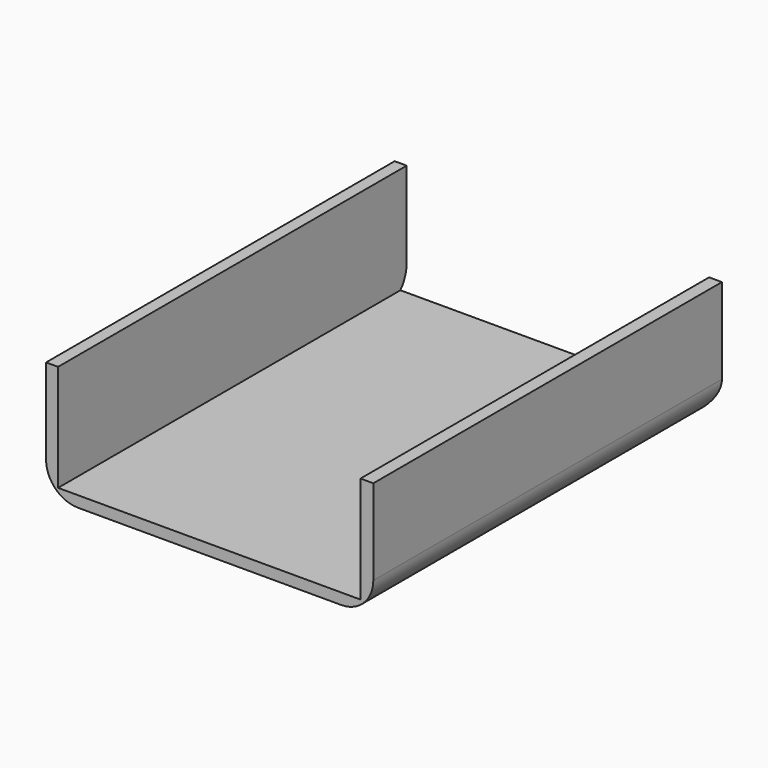
from build123d import *

# Parameters (mm, degrees)
F1_DEPTH    = 34.52499953
F2_T1_DEPTH = 94.44999906
F2_T3_DEPTH = 77.25000044


# Not quite as in the source:
# - a fillet or chamfer that OpenCascade refuses, or shapes differently, is made with other operations: its cross-section is extruded or revolved along the edge and cut away or added


with BuildPart() as f1:
    # F0 (on Front) → F1 (new body, symmetric)
    with BuildSketch(Plane.XZ):
        Polygon((-24.9640439777, 0), (-24.9640439777, -18.630000078), (26.8859564623, -18.630000078), (26.8859564623, 0), (24.8539564623, 0), (24.8539564623, -16.881729), (-23.0624323377, -16.881729), (-23.0624323377, 0), align=None)
    extrude(amount=F1_DEPTH, both=True)

    # F2: fillet of radius 5.08 on 3 edges, made by hand

    # F2_s2 → F2_t1 (cut)
    with BuildSketch(Plane.XZ.offset(-47.22499953)):
        with BuildLine():
            ThreePointArc((26.8859564623, -13.550000078), (25.3980589107, -17.1421025264), (21.8059564623, -18.630000078))
            Line((21.8059564623, -18.630000078), (26.8859564623, -18.630000078))
            Line((26.8859564623, -18.630000078), (26.8859564623, -13.550000078))
        make_face()
        with BuildLine():
            ThreePointArc((-24.9640439777, -13.550000078), (-23.4761464261, -17.1421025264), (-19.8840439777, -18.630000078))
            Line((-19.8840439777, -18.630000078), (-24.9640439777, -18.630000078))
            Line((-24.9640439777, -18.630000078), (-24.9640439777, -13.550000078))
        make_face()
    extrude(amount=F2_T1_DEPTH, mode=Mode.SUBTRACT)

    # F2_s4 → F2_t3 (cut)
    with BuildSketch(Plane.YZ.offset(-37.6640439777)):
        with BuildLine():
            ThreePointArc((29.44499953, -18.630000078), (33.0371019784, -17.1421025264), (34.52499953, -13.550000078))
            Line((34.52499953, -13.550000078), (34.52499953, -18.630000078))
            Line((34.52499953, -18.630000078), (29.44499953, -18.630000078))
        make_face()
    extrude(amount=F2_T3_DEPTH, mode=Mode.SUBTRACT)


solid = f1.part
